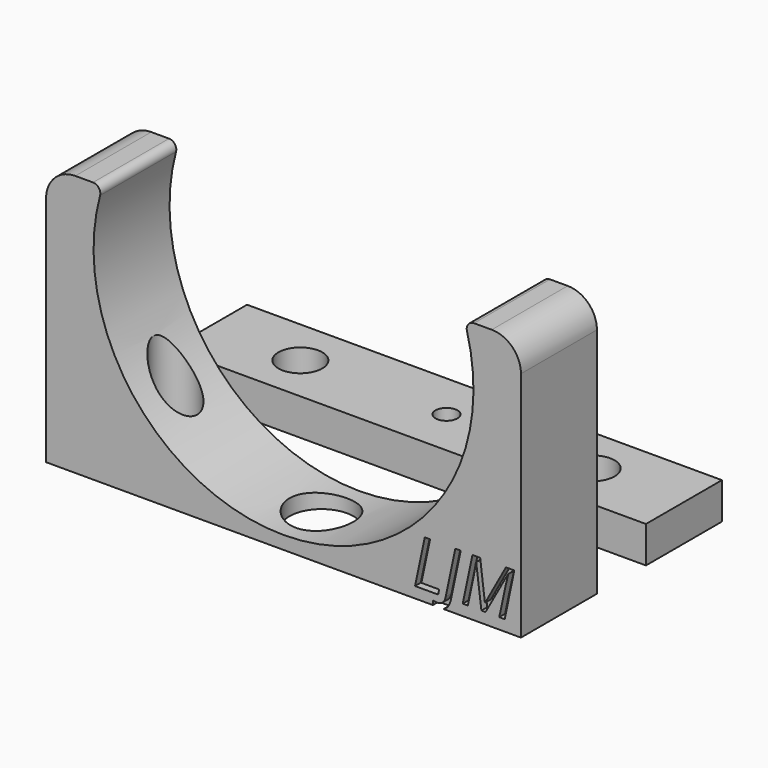
from build123d import *

# Parameters (mm, degrees)
F2_DEPTH     = 6.5
F1_R         = 4.375
F1_R_2       = 1.875
F3_DEPTH     = 27.801
F4_R         = 3
F4_W         = 65
F4_H         = 13
F4_R_2       = 1.5
F5_DEPTH     = 25
F4_R_3       = 1.875
F6_DEPTH     = 2.5
F7_TEXT_SIZE = 8.8302754901
F8_DEPTH     = 1
F9_DEPTH     = 5


# Not quite as in the source:
# - Text() gives the source's letters only with a copy of the font that has no kerning and outlines rounded to 1/6400 em; it was checked with that copy


with BuildPart() as f2:
    # F0 (on Front) → F2 (new body, symmetric)
    with BuildSketch(Plane.XZ):
        with BuildLine():
            Line((-32.5, -27.8), (32.5, -27.8))
            Line((32.5, -27.8), (32.5, 4))
            ThreePointArc((32.5, 4), (31.3284271247, 6.8284271247), (28.5, 8))
            Line((28.5, 8), (26.0768096208, 8))
            ThreePointArc((26.0768096208, 8), (25.2833175732, 7.6085806195), (25.1110018571, 6.7407407407))
            ThreePointArc((25.1110018571, 6.7407407407), (0, -26), (-25.1110018571, 6.7407407407))
            ThreePointArc((-25.1110018571, 6.7407407407), (-25.2833175732, 7.6085806195), (-26.0768096208, 8))
            Line((-26.0768096208, 8), (-28.5, 8))
            ThreePointArc((-28.5, 8), (-31.3284271247, 6.8284271247), (-32.5, 4))
            Line((-32.5, 4), (-32.5, -27.8))
        make_face()
    extrude(amount=F2_DEPTH, both=True)

    # F1 (on Top) → F3 (cut, through all)
    with BuildSketch(Plane.XY):
        Circle(F1_R)
        with Locations((20, 0)):
            Circle(F1_R_2)
        with Locations((-20, 0)):
            Circle(F1_R_2)
    extrude(amount=-F3_DEPTH, mode=Mode.SUBTRACT)

    # F4 (on face) → F5 (cut)
    with BuildSketch(Plane(origin=(0, 0, -27.8), x_dir=(1, 0, 0), z_dir=(0, 0, -1))):
        with Locations((20, 0)):
            Circle(F4_R)
        with Locations((-20, 0)):
            Circle(F4_R)
        with Locations((0, -21.3853213936)):
            Rectangle(F4_W, F4_H)
        with Locations((-20, -21.3853213936)):
            Circle(F4_R, mode=Mode.SUBTRACT)
        with Locations((0, -21.3853213936)):
            Circle(F4_R_2, mode=Mode.SUBTRACT)
        with Locations((20, -21.3853213936)):
            Circle(F4_R, mode=Mode.SUBTRACT)
    extrude(amount=-F5_DEPTH, mode=Mode.SUBTRACT)

    # F4 (on face) → F6 (join)
    with BuildSketch(Plane(origin=(0, 0, -27.8), x_dir=(1, 0, 0), z_dir=(0, 0, -1))):
        with Locations((20, 0)):
            Circle(F4_R)
        with Locations((20, 0)):
            Circle(F4_R_3, mode=Mode.SUBTRACT)
        with Locations((-20, 0)):
            Circle(F4_R)
        with Locations((-20, 0)):
            Circle(F4_R_3, mode=Mode.SUBTRACT)
    extrude(amount=-F6_DEPTH)

    # F7 (on face) → F8 (cut)
    with BuildSketch(Plane.XZ.offset(6.5)):
        with Locations((17.6284424961, -26.298167184)):
            Text('LJM', F7_TEXT_SIZE, font='Open Sans', font_style=FontStyle.ITALIC, text_align=(TextAlign.LEFT, TextAlign.BOTTOM))
    extrude(amount=-F8_DEPTH, mode=Mode.SUBTRACT)


with BuildPart() as f9:
    # F4 (on face) → F9 (new body)
    with BuildSketch(Plane(origin=(0, 0, -27.8), x_dir=(1, 0, 0), z_dir=(0, 0, -1))):
        with Locations((0, -21.3853213936)):
            Rectangle(F4_W, F4_H)
        with Locations((-20, -21.3853213936)):
            Circle(F4_R, mode=Mode.SUBTRACT)
        with Locations((0, -21.3853213936)):
            Circle(F4_R_2, mode=Mode.SUBTRACT)
        with Locations((20, -21.3853213936)):
            Circle(F4_R, mode=Mode.SUBTRACT)
    extrude(amount=-F9_DEPTH)


solid = Compound([f2.part, f9.part])
